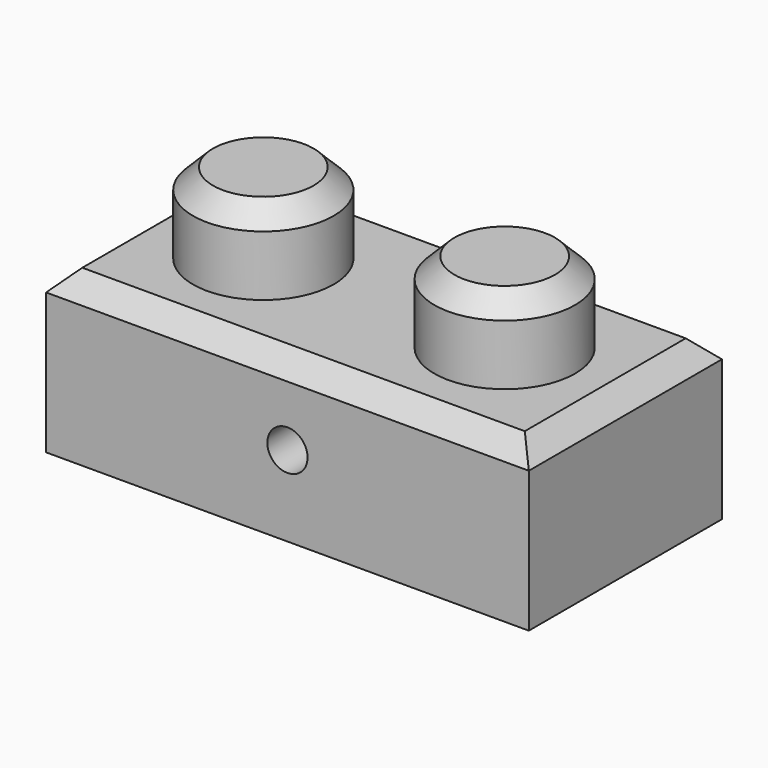
from build123d import *

# Parameters (mm, degrees)
F0_W     = 76.2
F0_H     = 38.1
F1_DEPTH = 25.4
F2_R     = 11.1125
F3_DEPTH = 12.7
F4_SIZE  = 3.175
F5_T     = 7.9375
F6_R     = 3.175
F7_DEPTH = 7.9375
F8_R     = 3.0126564395
F9_DEPTH = 7.9375


# Not quite as in the source:
# - a shell that OpenCascade refuses in one call is made with other operations: the cavity is built on its own and cut out


with BuildPart() as f1:
    # F0 (on Top) → F1 (new body)
    with BuildSketch(Plane.XY):
        with Locations((-5.8783623338, 3.9097142845)):
            Rectangle(F0_W, F0_H)
    extrude(amount=F1_DEPTH)

    # F2 (on face) → F3 (join)
    with BuildSketch(Plane.XY.offset(25.4)):
        with Locations((-24.9283623338, 3.9097142845)):
            Circle(F2_R)
        with Locations((13.1716376662, 3.9097142845)):
            Circle(F2_R)
    extrude(amount=F3_DEPTH)

    # F4
    f4_edges = [f1.edges().sort_by_distance(p)[0] for p in [
        (-36.040862, 3.909714, 38.1),
        (2.059138, 3.909714, 38.1),
        (32.221638, 3.909714, 25.4),
        (-5.878362, 22.959714, 25.4),
        (-43.978362, 3.909714, 25.4),
        (-5.878362, -15.140286, 25.4),
    ]]
    chamfer(f4_edges, length=F4_SIZE)

    # F5: shell of thickness 7.9375, made by hand


with BuildPart() as f5_core1:
    # F5_t2: copy of F1
    add(f1.part)

    # the walls: a layer under each face that stays
    f5_faces = [f5_core1.faces().sort_by_distance(p)[0] for p in [
        (32.2216376662, 3.9097142845, 11.1125),
        (-5.8783623338, -15.1402857155, 11.1125),
        (30.6341376662, 3.9097142845, 23.8125),
        (-5.8783623338, 22.9597142845, 11.1125),
        (-43.9783623338, 3.9097142845, 11.1125),
        (-5.8783623338, -13.5527857155, 23.8125),
        (-5.8783623338, 3.9097142845, 25.4),
        (-5.8783623338, 21.3722142845, 23.8125),
        (-42.3908623338, 3.9097142845, 23.8125),
        (-36.0408623338, 3.9097142845, 30.1625),
        (2.0591376662, 3.9097142845, 30.1625),
        (-34.4533623338, 3.9097142845, 36.5125),
        (3.6466376662, 3.9097142845, 36.5125),
        (-24.9283623338, 3.9097142845, 38.1),
        (13.1716376662, 3.9097142845, 38.1),
    ]]
    thicken(f5_faces, amount=-F5_T, mode=Mode.SUBTRACT)

    # F5_s3 → F5_t4 (revolve, cut)
    with BuildSketch(Plane.XZ.offset(-3.9097142845)):
        Polygon((-13.7364873338, 25.479375), (-13.8158623338, 17.4625), (-21.7533623338, 17.4625), (-21.7533623338, 25.4), align=None)
    revolve(axis=Axis((-24.9283623338, 3.9097142845, 25.4), (0, 0, 1)), mode=Mode.SUBTRACT)

    # F5_s5 → F5_t6 (revolve, cut)
    with BuildSketch(Plane.XZ.offset(-3.9097142845)):
        Polygon((24.3635126662, 25.479375), (24.2841376662, 17.4625), (16.3466376662, 17.4625), (16.3466376662, 25.4), align=None)
    revolve(axis=Axis((13.1716376662, 3.9097142845, 25.4), (0, 0, 1)), mode=Mode.SUBTRACT)


with BuildPart() as f1_1:
    add(f1.part)

    # what is left inside the walls is the cavity
    f5_cavity = [f5_core1.part.solids().sort_by_distance(p)[0] for p in [
        (-5.878362, 0.205548, 0.079375),
    ]]
    add(f5_cavity, mode=Mode.SUBTRACT)

    # F6 (on face) → F7 (cut)
    with BuildSketch(Plane.XZ.offset(15.1402857155)):
        with Locations((-5.8783623338, 12.7)):
            Circle(F6_R)
    extrude(amount=-F7_DEPTH, mode=Mode.SUBTRACT)

    # F8 (on face) → F9 (cut)
    with BuildSketch(Plane(origin=(0, 22.9597142845, 0), x_dir=(-1, 0, 0), z_dir=(0, 1, 0))):
        with Locations((5.8783623338, 12.7)):
            Circle(F8_R)
    extrude(amount=-F9_DEPTH, mode=Mode.SUBTRACT)


solid = f1_1.part
